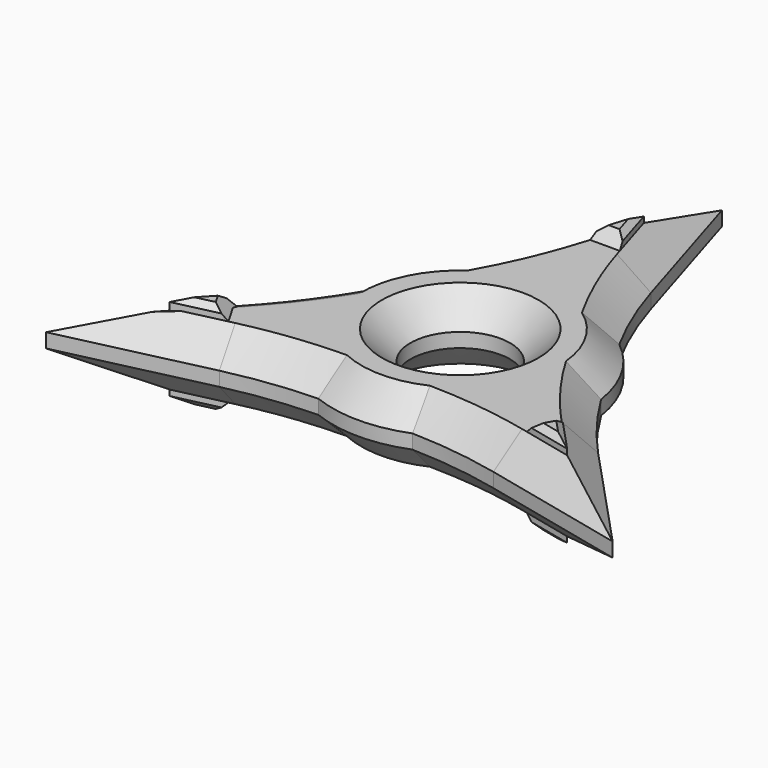
from build123d import *

# Parameters (mm, degrees)
F1_DEPTH      = 12.5
F2_R          = 8.722464072
F3_DEPTH      = 25
F4_C1_SIZE    = 5
F4_C2_SIZE    = 5
F4_C3_SIZE    = 5
F4_C4_SIZE    = 5
F4_C5_SIZE    = 5
F4_C6_SIZE    = 5
F4_C7_SIZE    = 5
F4_C8_SIZE    = 5
F4_C9_SIZE    = 5
F4_C10_SIZE   = 5
F4_C11_SIZE   = 5
F4_C12_SIZE   = 5
F4_C13_SIZE   = 5
F4_C14_SIZE   = 5
F4_C15_SIZE   = 4.9999
F4_C16_SIZE   = 4.9999
F4_C17_SIZE   = 4.9999
F4_C18_SIZE   = 4.9999
F6_DEPTH      = 2
F6_DEPTH_BACK = 14.5
F7_SIZE       = 1
F7_2_SIZE     = 1
F7_3_SIZE     = 1
F7_4_SIZE     = 1
F8_SIZE       = 1
F9_SIZE       = 5
F10_SIZE      = 3
F10_2_SIZE    = 3
F10_3_SIZE    = 3


# Not quite as in the source:
# - a fillet or chamfer is up to 0.001 mm smaller than in the source, because OpenCascade refuses the exact size


with BuildPart() as f1:
    # F0 (on Top) → F1 (new body)
    with BuildSketch(Plane.XY):
        with BuildLine():
            ThreePointArc((-8.2462994883, -20.746848224), (-19.3345513229, -11.162808411), (-22.0904473546, 3.2319192679))
            ThreePointArc((-22.0904473546, 3.2319192679), (-26.5638124389, -3.3325951278), (-31.6795363045, -9.4098653834))
            Line((-31.6795363045, -9.4098653834), (-49.6173238599, -28.646575287))
            Line((-49.6173238599, -28.646575287), (-23.9889506205, -22.7303505281))
            ThreePointArc((-23.9889506205, -22.7303505281), (-16.1680182607, -21.3386388295), (-8.2462994883, -20.746848224))
        make_face()
        with BuildLine():
            ThreePointArc((-7.690585684, 32.1402159115), (-10.3957941782, 24.6712339574), (-13.8441478662, 17.5149289561))
            ThreePointArc((-13.8441478662, 17.5149289561), (-19.3345513229, 11.162808411), (-22.0904473546, 3.2319192679))
            ThreePointArc((-22.0904473546, 3.2319192679), (-19.3345513229, -11.162808411), (-8.2462994883, -20.746848224))
            ThreePointArc((-8.2462994883, -20.746848224), (0, -22.3256168219), (8.2462994883, -20.746848224))
            ThreePointArc((8.2462994883, -20.746848224), (19.3345513229, -11.162808411), (22.0904473546, 3.2319192679))
            ThreePointArc((22.0904473546, 3.2319192679), (19.3345513229, 11.162808411), (13.8441478662, 17.5149289561))
            ThreePointArc((13.8441478662, 17.5149289561), (10.3957941782, 24.6712339574), (7.690585684, 32.1402159115))
            Line((7.690585684, 32.1402159115), (0, 57.293150574))
            Line((0, 57.293150574), (-7.690585684, 32.1402159115))
        make_face()
        with BuildLine():
            ThreePointArc((22.0904473546, 3.2319192679), (19.3345513229, -11.162808411), (8.2462994883, -20.746848224))
            ThreePointArc((8.2462994883, -20.746848224), (16.1680182607, -21.3386388295), (23.9889506205, -22.7303505281))
            Line((23.9889506205, -22.7303505281), (49.6173238599, -28.646575287))
            Line((49.6173238599, -28.646575287), (31.6795363045, -9.4098653834))
            ThreePointArc((31.6795363045, -9.4098653834), (26.5638124389, -3.3325951278), (22.0904473546, 3.2319192679))
        make_face()
    extrude(amount=F1_DEPTH)

    # F2 (on face) → F3 (cut)
    with BuildSketch(Plane.XY.offset(12.5)):
        Circle(F2_R)
    extrude(amount=-F3_DEPTH, mode=Mode.SUBTRACT)

    # F4: chamfer of 5 on 18 edges, made by hand

    # F4_c1
    f4_c1_edges = [f1.edges().sort_by_distance(p)[0] for p in [
        (-16.1680182607, -21.3386388295, 0),
        (-36.8031372402, -25.6884629075, 0),
    ]]
    chamfer(f4_c1_edges, length=F4_C1_SIZE)

    # F4_c2
    f4_c2_edges = [f1.edges().sort_by_distance(p)[0] for p in [
        (-16.1680182607, -21.3386388295, 12.5),
        (-36.8031372402, -25.6884629075, 12.5),
    ]]
    chamfer(f4_c2_edges, length=F4_C2_SIZE)

    # F4_c3
    f4_c3_edges = [f1.edges().sort_by_distance(p)[0] for p in [
        (-37.5996515992, -15.7586717882, 0),
        (-26.5638124389, -3.3325951278, 0),
    ]]
    chamfer(f4_c3_edges, length=F4_C3_SIZE)

    # F4_c4
    f4_c4_edges = [f1.edges().sort_by_distance(p)[0] for p in [
        (16.1680182607, -21.3386388295, 0),
        (36.8031372402, -25.6884629075, 0),
    ]]
    chamfer(f4_c4_edges, length=F4_C4_SIZE)

    # F4_c5
    f4_c5_edges = [f1.edges().sort_by_distance(p)[0] for p in [
        (37.5996515992, -15.7586717882, 0),
        (26.5638124389, -3.3325951278, 0),
    ]]
    chamfer(f4_c5_edges, length=F4_C5_SIZE)

    # F4_c6
    f4_c6_edges = [f1.edges().sort_by_distance(p)[0] for p in [
        (-10.3957941782, 24.6712339574, 0),
        (-3.845292842, 44.7166832427, 0),
    ]]
    chamfer(f4_c6_edges, length=F4_C6_SIZE)

    # F4_c7
    f4_c7_edges = [f1.edges().sort_by_distance(p)[0] for p in [
        (5.1524157011, 40.4415893525, 0),
        (10.3957941782, 24.6712339574, 0),
    ]]
    chamfer(f4_c7_edges, length=F4_C7_SIZE)

    # F4_c8
    f4_c8_edges = [f1.edges().sort_by_distance(p)[0] for p in [
        (-37.5996515992, -15.7586717882, 12.5),
        (-26.5638124389, -3.3325951278, 12.5),
    ]]
    chamfer(f4_c8_edges, length=F4_C8_SIZE)

    # F4_c9
    f4_c9_edges = [f1.edges().sort_by_distance(p)[0] for p in [
        (16.1680182607, -21.3386388295, 12.5),
        (36.8031372402, -25.6884629075, 12.5),
    ]]
    chamfer(f4_c9_edges, length=F4_C9_SIZE)

    # F4_c10
    f4_c10_edges = [f1.edges().sort_by_distance(p)[0] for p in [
        (37.5996515992, -15.7586717882, 12.5),
        (26.5638124389, -3.3325951278, 12.5),
    ]]
    chamfer(f4_c10_edges, length=F4_C10_SIZE)

    # F4_c11
    f4_c11_edges = [f1.edges().sort_by_distance(p)[0] for p in [
        (-10.3957941782, 24.6712339574, 12.5),
        (-3.845292842, 44.7166832427, 12.5),
    ]]
    chamfer(f4_c11_edges, length=F4_C11_SIZE)

    # F4_c12
    f4_c12_edges = [f1.edges().sort_by_distance(p)[0] for p in [
        (5.1524157011, 40.4415893525, 12.5),
        (10.3957941782, 24.6712339574, 12.5),
    ]]
    chamfer(f4_c12_edges, length=F4_C12_SIZE)

    # F4_c13
    f4_c13_edges = [f1.edges().sort_by_distance(p)[0] for p in [
        (0, -22.3256168219, 0),
    ]]
    chamfer(f4_c13_edges, length=F4_C13_SIZE)

    # F4_c14
    f4_c14_edges = [f1.edges().sort_by_distance(p)[0] for p in [
        (0, -22.3256168219, 12.5),
    ]]
    chamfer(f4_c14_edges, length=F4_C14_SIZE)

    # F4_c15 (size 5 in the source; OpenCascade refuses exactly that, so slightly less here)
    f4_c15_edges = [f1.edges().sort_by_distance(p)[0] for p in [
        (-19.3345513229, 11.162808411, 0),
    ]]
    chamfer(f4_c15_edges, length=F4_C15_SIZE)

    # F4_c16 (size 5 in the source; OpenCascade refuses exactly that, so slightly less here)
    f4_c16_edges = [f1.edges().sort_by_distance(p)[0] for p in [
        (19.3345513229, 11.162808411, 0),
    ]]
    chamfer(f4_c16_edges, length=F4_C16_SIZE)

    # F4_c17 (size 5 in the source; OpenCascade refuses exactly that, so slightly less here)
    f4_c17_edges = [f1.edges().sort_by_distance(p)[0] for p in [
        (-19.3345513229, 11.162808411, 12.5),
    ]]
    chamfer(f4_c17_edges, length=F4_C17_SIZE)

    # F4_c18 (size 5 in the source; OpenCascade refuses exactly that, so slightly less here)
    f4_c18_edges = [f1.edges().sort_by_distance(p)[0] for p in [
        (19.3345513229, 11.162808411, 12.5),
    ]]
    chamfer(f4_c18_edges, length=F4_C18_SIZE)

    # F7#4
    f7_4_edges = [f1.edges().sort_by_distance(p)[0] for p in [
        (-31.415331, -16.458085, 12.5),
    ]]
    chamfer(f7_4_edges, length=F7_4_SIZE)

    # F9
    f9_edges = [f1.edges().sort_by_distance(p)[0] for p in [
        (-8.722464, 0, 12.5),
        (-8.722464, 0, 0),
    ]]
    chamfer(f9_edges, length=F9_SIZE)


with BuildPart() as f6:
    # F5 (on face) → F6 (new body, two sides)
    with BuildSketch(Plane(origin=(0, 0, 0), x_dir=(1, 0, 0), z_dir=(0, 0, -1))) as f6_sk:
        Polygon((-28.0226981411, 12.8197824861), (-25.1136063745, 17.8584772298), (-34.8079642097, 20.0963875064), align=None)
    extrude(amount=F6_DEPTH)
    extrude(f6_sk.sketch, amount=-F6_DEPTH_BACK)

    # F7#2
    f7_2_edges = [f6.edges().sort_by_distance(p)[0] for p in [
        (-29.960785, -18.977432, -2),
        (-31.415331, -16.458085, -2),
        (-29.960785, -18.977432, 14.5),
    ]]
    chamfer(f7_2_edges, length=F7_2_SIZE)

    # F8
    f8_edges = [f6.edges().sort_by_distance(p)[0] for p in [
        (-30.805575, -15.804175, 14.5),
    ]]
    chamfer(f8_edges, length=F8_SIZE)

    # F10#2
    f10_2_edges = [f6.edges().sort_by_distance(p)[0] for p in [
        (-26.568152, -15.33913, 14.5),
        (-26.568152, -15.33913, -2),
    ]]
    chamfer(f10_2_edges, length=F10_2_SIZE)


with BuildPart() as f6b:
    # F5 (on face) → F6, piece 2 (new body, two sides)
    with BuildSketch(Plane(origin=(0, 0, 0), x_dir=(1, 0, 0), z_dir=(0, 0, -1))) as f6_2_sk:
        Polygon((0, -40.1927750129), (2.9090917667, -30.6782597158), (-2.9090917667, -30.6782597158), align=None)
    extrude(amount=F6_DEPTH)
    extrude(f6_2_sk.sketch, amount=-F6_DEPTH_BACK)

    # F7#3
    f7_3_edges = [f6b.edges().sort_by_distance(p)[0] for p in [
        (1.454546, 35.435517, -2),
        (-1.454546, 35.435517, -2),
        (1.454546, 35.435517, 14.5),
        (-1.454546, 35.435517, 14.5),
    ]]
    chamfer(f7_3_edges, length=F7_3_SIZE)

    # F10
    f10_edges = [f6b.edges().sort_by_distance(p)[0] for p in [
        (0, 30.67826, -2),
        (0, 30.67826, 14.5),
    ]]
    chamfer(f10_edges, length=F10_SIZE)


with BuildPart() as f6c:
    # F5 (on face) → F6, piece 3 (new body, two sides)
    with BuildSketch(Plane(origin=(0, 0, 0), x_dir=(1, 0, 0), z_dir=(0, 0, -1))) as f6_3_sk:
        Polygon((28.0226981411, 12.8197824861), (34.8079642097, 20.0963875064), (25.1136063745, 17.8584772298), align=None)
    extrude(amount=F6_DEPTH)
    extrude(f6_3_sk.sketch, amount=-F6_DEPTH_BACK)

    # F7
    f7_edges = [f6c.edges().sort_by_distance(p)[0] for p in [
        (29.960785, -18.977432, -2),
        (31.415331, -16.458085, -2),
        (31.415331, -16.458085, 14.5),
        (29.960785, -18.977432, 14.5),
    ]]
    chamfer(f7_edges, length=F7_SIZE)

    # F10#3
    f10_3_edges = [f6c.edges().sort_by_distance(p)[0] for p in [
        (26.568152, -15.33913, 14.5),
        (26.568152, -15.33913, -2),
    ]]
    chamfer(f10_3_edges, length=F10_3_SIZE)


solid = Compound([f1.part, f6.part, f6b.part, f6c.part])
